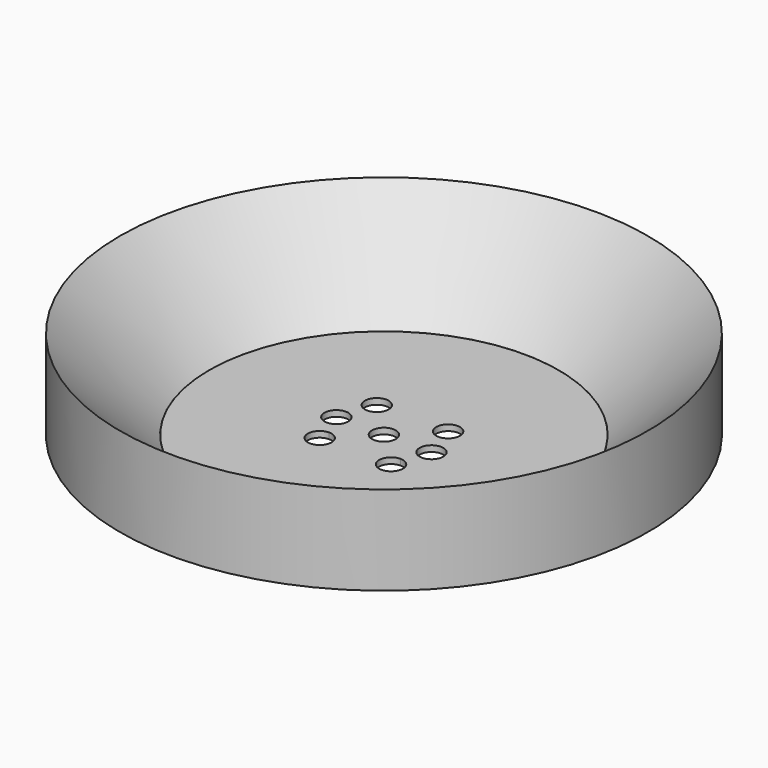
from build123d import *

# Parameters (mm, degrees)
F2_R     = 20
F5_DEPTH = 10


# Not quite as in the source:
# - the program builds the solid bodies; features that only make, move or delete a surface that nothing else refers to are left out


with BuildPart() as f1:
    # F0 (on Front) → F1 (revolve)
    with BuildSketch(Plane.XZ):
        Polygon((-444, 300), (-444, 150), (-294, 150), align=None)
    revolve(axis=Axis((0, 0, 272.4012136459), (0, 0, 1)))


with BuildPart() as f5:
    # F2 (on face) → F5 (new body)
    with BuildSketch(Plane(origin=(0, 0, 150), x_dir=(1, 0, 0), z_dir=(0, 0, -1))):
        Polygon((249.8219365868, 155), (0, 155), (-249.8219365868, 155), (0, -294), align=None)
        Polygon((-203.0846477822, 125), (0, 125), (203.0846477822, 125), (0, -240), align=None, mode=Mode.SUBTRACT)
        Polygon((203.0846477822, 125), (0, 125), (-203.0846477822, 125), (0, -240), align=None)
        with BuildLine():
            ThreePointArc((-40, -60), (-74.1421356237, -74.1421356237), (-60, -40))
            ThreePointArc((-60, -40), (-45.8578643763, -45.8578643763), (-40, -60))
        make_face(mode=Mode.SUBTRACT)
        with BuildLine():
            ThreePointArc((80, -60), (45.8578643763, -74.1421356237), (60, -40))
            ThreePointArc((60, -40), (74.1421356237, -45.8578643763), (80, -60))
        make_face(mode=Mode.SUBTRACT)
        with Locations((-80, 0)):
            Circle(F2_R, mode=Mode.SUBTRACT)
        with BuildLine():
            ThreePointArc((-40, 60), (-45.8578643763, 45.8578643763), (-60, 40))
            ThreePointArc((-60, 40), (-74.1421356237, 74.1421356237), (-40, 60))
        make_face(mode=Mode.SUBTRACT)
        with BuildLine():
            ThreePointArc((-20, 0), (0, 20), (20, 0))
            ThreePointArc((20, 0), (0, -20), (-20, 0))
        make_face(mode=Mode.SUBTRACT)
        with BuildLine():
            ThreePointArc((100, 0), (79.9999999661, -20), (60, 6.79e-08))
            ThreePointArc((60, 6.79e-08), (80.0000000339, 20), (100, 0))
        make_face(mode=Mode.SUBTRACT)
        with BuildLine():
            ThreePointArc((80, 60), (74.1421356237, 45.8578643763), (60, 40))
            ThreePointArc((60, 40), (45.8578643763, 74.1421356237), (80, 60))
        make_face(mode=Mode.SUBTRACT)
        with BuildLine():
            Line((0, -294), (-249.8219365868, 155))
            ThreePointArc((-249.8219365868, 155), (-256.910490249, -142.9440449966), (0, -294))
        make_face()
        with BuildLine():
            ThreePointArc((294, 0), (282.7398533604, 80.5864462657), (249.8219365868, 155))
            Line((249.8219365868, 155), (0, -294))
            ThreePointArc((0, -294), (207.8893936688, -207.8893936688), (294, 0))
        make_face()
        with BuildLine():
            Line((-249.8219365868, 155), (0, 155))
            Line((0, 155), (249.8219365868, 155))
            ThreePointArc((249.8219365868, 155), (0, 294), (-249.8219365868, 155))
        make_face()
    extrude(amount=F5_DEPTH)


solid = Compound([f1.part, f5.part])
